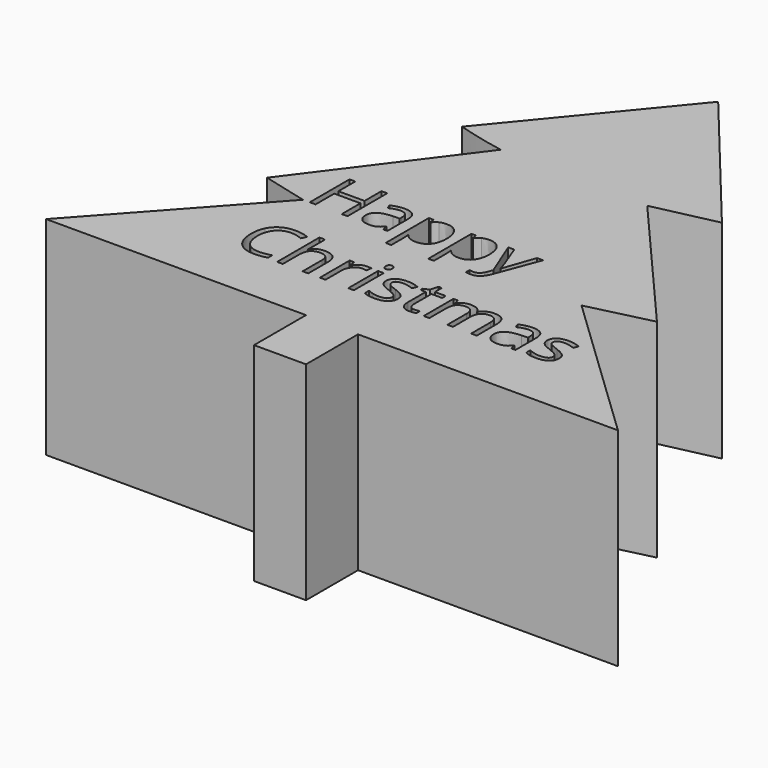
from build123d import *

# Parameters (mm, degrees)
F1_DEPTH = 6.95914
F2_W     = 0.8686156983
F2_H     = 5.7321941552
F3_DEPTH = 25


with BuildPart() as f1:
    # F0 (on Top) → F1 (new body)
    with BuildSketch(Plane.XY):
        with BuildLine():
            Line((-12.3236204717, 43.3583846717), (-32.2978136329, 19.0763476119))
            Line((-32.2978136329, 19.0763476119), (-12.2978136329, 19.0763476119))
            Line((-12.2978136329, 19.0763476119), (-12.2978136329, 43.3583799146))
            ThreePointArc((-12.2978136329, 43.3583799146), (-12.3107170525, 43.3583811039), (-12.3236204717, 43.3583846717))
        make_face()
        Polygon((-12.2978136329, 43.3583799146), (-12.2978136329, 19.0763476119), (7.7021863671, 19.0763476119), align=None)
        with BuildLine():
            ThreePointArc((-32.2978136329, 19.0763476119), (-28.6304707138, 18.0904479885), (-24.9150584445, 17.3048820634))
            ThreePointArc((-24.9150584445, 17.3048820634), (-18.6324272302, 16.4455999422), (-12.2978136329, 16.1583869369))
            Line((-12.2978136329, 16.1583869369), (-12.2978136329, 19.0763476119))
            Line((-12.2978136329, 19.0763476119), (-32.2978136329, 19.0763476119))
        make_face()
        with BuildLine():
            Line((-12.2978136329, 19.0763476119), (-12.2978136329, 16.1583869369))
            ThreePointArc((-12.2978136329, 16.1583869369), (-7.1653753165, 16.3467970901), (-2.0605656712, 16.9110133104))
            Line((-2.0605656712, 16.9110133104), (7.7021863671, 19.0763476119))
            Line((7.7021863671, 19.0763476119), (-12.2978136329, 19.0763476119))
        make_face()
        with BuildLine():
            Line((-24.9150584445, 17.3048820634), (-42.2978136329, -5.9236523881))
            Line((-42.2978136329, -5.9236523881), (-12.2978136329, -5.9236523881))
            Line((-12.2978136329, -5.9236523881), (-12.2978136329, 16.1583869369))
            ThreePointArc((-12.2978136329, 16.1583869369), (-18.6324272302, 16.4455999422), (-24.9150584445, 17.3048820634))
        make_face()
        with BuildLine():
            Line((-12.2978136329, 16.1583869369), (-12.2978136329, -5.9236523881))
            Line((-12.2978136329, -5.9236523881), (17.7021863671, -5.9236523881))
            Line((17.7021863671, -5.9236523881), (-2.0605656712, 16.9110133104))
            ThreePointArc((-2.0605656712, 16.9110133104), (-7.1653753165, 16.3467970901), (-12.2978136329, 16.1583869369))
        make_face()
        with BuildLine():
            Line((-42.2978136329, -5.9236523881), (-35.339471558, -7.7121023845))
            ThreePointArc((-35.339471558, -7.7121023845), (-23.8873413462, -9.60026092), (-12.2978136329, -10.2321441568))
            Line((-12.2978136329, -10.2321441568), (-12.2978136329, -5.9236523881))
            Line((-12.2978136329, -5.9236523881), (-42.2978136329, -5.9236523881))
        make_face()
        with BuildLine():
            Line((-12.2978136329, -5.9236523881), (-12.2978136329, -10.2321441568))
            ThreePointArc((-12.2978136329, -10.2321441568), (-2.1098095313, -9.7441780676), (7.9849217698, -8.2847472074))
            Line((7.9849217698, -8.2847472074), (17.7021863671, -5.9236523881))
            Line((17.7021863671, -5.9236523881), (-12.2978136329, -5.9236523881))
        make_face()
        with BuildLine():
            Line((-56.2978136329, -30.9236523881), (-16.2978136329, -30.9236523881))
            Line((-16.2978136329, -30.9236523881), (-12.2978136329, -30.9236523881))
            Line((-12.2978136329, -30.9236523881), (-12.2978136329, -10.2321441568))
            ThreePointArc((-12.2978136329, -10.2321441568), (-23.8873413462, -9.60026092), (-35.339471558, -7.7121023845))
            Line((-35.339471558, -7.7121023845), (-56.2978136329, -30.9236523881))
        make_face()
        with BuildLine():
            Line((-12.2978136329, -30.9236523881), (-8.2978136329, -30.9236523881))
            Line((-8.2978136329, -30.9236523881), (31.7021863671, -30.9236523881))
            Line((31.7021863671, -30.9236523881), (7.9849217698, -8.2847472074))
            ThreePointArc((7.9849217698, -8.2847472074), (-2.1098095313, -9.7441780676), (-12.2978136329, -10.2321441568))
            Line((-12.2978136329, -10.2321441568), (-12.2978136329, -30.9236523881))
        make_face()
        Polygon((-16.2978136329, -30.9236523881), (-16.2978136329, -40.9236523881), (-8.2978136329, -40.9236523881), (-8.2978136329, -30.9236523881), (-12.2978136329, -30.9236523881), align=None)
    extrude(amount=F1_DEPTH)

    # F2 (on face) → F3 (join)
    with BuildSketch(Plane.XY.offset(6.95914)):
        with BuildLine():
            Line((-2.0605656712, 16.9110133104), (7.7021863671, 19.0763476119))
            Line((7.7021863671, 19.0763476119), (-12.2978136329, 43.3583799146))
            ThreePointArc((-12.2978136329, 43.3583799146), (-12.3107170525, 43.3583811039), (-12.3236204717, 43.3583846717))
            Line((-12.3236204717, 43.3583846717), (-32.2978136329, 19.0763476119))
            ThreePointArc((-32.2978136329, 19.0763476119), (-28.6304707138, 18.0904479885), (-24.9150584445, 17.3048820634))
            Line((-24.9150584445, 17.3048820634), (-42.2978136329, -5.9236523881))
            Line((-42.2978136329, -5.9236523881), (-35.339471558, -7.7121023845))
            Line((-35.339471558, -7.7121023845), (-56.2978136329, -30.9236523881))
            Line((-56.2978136329, -30.9236523881), (-16.2978136329, -30.9236523881))
            Line((-16.2978136329, -30.9236523881), (-16.2978136329, -40.9236523881))
            Line((-16.2978136329, -40.9236523881), (-8.2978136329, -40.9236523881))
            Line((-8.2978136329, -40.9236523881), (-8.2978136329, -30.9236523881))
            Line((-8.2978136329, -30.9236523881), (31.7021863671, -30.9236523881))
            Line((31.7021863671, -30.9236523881), (7.9849217698, -8.2847472074))
            Line((7.9849217698, -8.2847472074), (17.7021863671, -5.9236523881))
            Line((17.7021863671, -5.9236523881), (-2.0605656712, 16.9110133104))
        make_face()
        with BuildLine():
            add(Edge.make_bspline(
                [(-29.2775716368, -15.7254587685), (-30.1461873351, -15.3187658693), (-31.0148030333, -15.3187658693)],
                knots=[0, 0, 0, 1, 1, 1], degree=2))
            add(Edge.make_bspline(
                [(-31.0148030333, -15.3187658693), (-32.2750489308, -15.3187658693), (-33.0047530627, -16.1580929843)],
                knots=[0, 0, 0, 1, 1, 1], degree=2))
            add(Edge.make_bspline(
                [(-33.0047530627, -16.1580929843), (-33.7344571945, -16.9974200992), (-33.7344571945, -18.456828363)],
                knots=[0, 0, 0, 1, 1, 1], degree=2))
            add(Edge.make_bspline(
                [(-33.7344571945, -18.456828363), (-33.7344571945, -19.9564038266), (-33.0306943793, -20.7756473417)],
                knots=[0, 0, 0, 1, 1, 1], degree=2))
            add(Edge.make_bspline(
                [(-33.0306943793, -20.7756473417), (-32.326931564, -21.5948908567), (-31.0248448333, -21.5948908567)],
                knots=[0, 0, 0, 1, 1, 1], degree=2))
            add(Edge.make_bspline(
                [(-31.0248448333, -21.5948908567), (-30.2248481016, -21.5948908567), (-29.1989108703, -21.3070259239)],
                knots=[0, 0, 0, 1, 1, 1], degree=2))
            Line((-29.1989108703, -21.3070259239), (-29.1989108703, -22.0852654224))
            add(Edge.make_bspline(
                [(-29.1989108703, -22.0852654224), (-29.993886702, -22.3848457884), (-31.160409133, -22.3848457884)],
                knots=[0, 0, 0, 1, 1, 1], degree=2))
            add(Edge.make_bspline(
                [(-31.160409133, -22.3848457884), (-32.849105163, -22.3848457884), (-33.7670930445, -21.3589085572)],
                knots=[0, 0, 0, 1, 1, 1], degree=2))
            add(Edge.make_bspline(
                [(-33.7670930445, -21.3589085572), (-34.685080926, -20.3329713259), (-34.685080926, -18.4451129297)],
                knots=[0, 0, 0, 1, 1, 1], degree=2))
            add(Edge.make_bspline(
                [(-34.685080926, -18.4451129297), (-34.685080926, -17.2635277987), (-34.2432417268, -16.3748285005)],
                knots=[0, 0, 0, 1, 1, 1], degree=2))
            add(Edge.make_bspline(
                [(-34.2432417268, -16.3748285005), (-33.8014025277, -15.4861292023), (-32.9670963127, -15.0049596199)],
                knots=[0, 0, 0, 1, 1, 1], degree=2))
            add(Edge.make_bspline(
                [(-32.9670963127, -15.0049596199), (-32.1327900977, -14.5237900375), (-31.0030876, -14.5237900375)],
                knots=[0, 0, 0, 1, 1, 1], degree=2))
            add(Edge.make_bspline(
                [(-31.0030876, -14.5237900375), (-29.8014188691, -14.5237900375), (-28.9010041375, -14.96228197)],
                knots=[0, 0, 0, 1, 1, 1], degree=2))
            Line((-28.9010041375, -14.96228197), (-29.2775716368, -15.7254587685))
        make_face(mode=Mode.SUBTRACT)
        with BuildLine():
            Line((-22.8692296163, -22.2794068887), (-23.7378453146, -22.2794068887))
            Line((-23.7378453146, -22.2794068887), (-23.7378453146, -18.5706354294))
            add(Edge.make_bspline(
                [(-23.7378453146, -18.5706354294), (-23.7378453146, -17.8710566975), (-24.0566724639, -17.5254514149)],
                knots=[0, 0, 0, 1, 1, 1], degree=2))
            add(Edge.make_bspline(
                [(-24.0566724639, -17.5254514149), (-24.3754996133, -17.1798461322), (-25.0566683786, -17.1798461322)],
                knots=[0, 0, 0, 1, 1, 1], degree=2))
            add(Edge.make_bspline(
                [(-25.0566683786, -17.1798461322), (-25.9604303768, -17.1798461322), (-26.3763282593, -17.6718943312)],
                knots=[0, 0, 0, 1, 1, 1], degree=2))
            add(Edge.make_bspline(
                [(-26.3763282593, -17.6718943312), (-26.7922261418, -18.1639425302), (-26.7922261418, -19.2819295947)],
                knots=[0, 0, 0, 1, 1, 1], degree=2))
            Line((-26.7922261418, -19.2819295947), (-26.7922261418, -22.2794068887))
            Line((-26.7922261418, -22.2794068887), (-27.66084184, -22.2794068887))
            Line((-27.66084184, -22.2794068887), (-27.66084184, -14.140528005))
            Line((-27.66084184, -14.140528005), (-26.7922261418, -14.140528005))
            Line((-26.7922261418, -14.140528005), (-26.7922261418, -16.6041162667))
            add(Edge.make_bspline(
                [(-26.7922261418, -16.6041162667), (-26.7922261418, -17.0493027325), (-26.834066975, -17.3421885652)],
                knots=[0, 0, 0, 1, 1, 1], degree=2))
            Line((-26.834066975, -17.3421885652), (-26.7821843418, -17.3421885652))
            add(Edge.make_bspline(
                [(-26.7821843418, -17.3421885652), (-26.5261184423, -16.9288011327), (-26.0524802099, -16.6911451999)],
                knots=[0, 0, 0, 1, 1, 1], degree=2))
            add(Edge.make_bspline(
                [(-26.0524802099, -16.6911451999), (-25.5788419775, -16.453489267), (-24.9729867121, -16.453489267)],
                knots=[0, 0, 0, 1, 1, 1], degree=2))
            add(Edge.make_bspline(
                [(-24.9729867121, -16.453489267), (-23.9219449809, -16.453489267), (-23.3955872986, -16.953068816)],
                knots=[0, 0, 0, 1, 1, 1], degree=2))
            add(Edge.make_bspline(
                [(-23.3955872986, -16.953068816), (-22.8692296163, -17.452648365), (-22.8692296163, -18.5405100295)],
                knots=[0, 0, 0, 1, 1, 1], degree=2))
            Line((-22.8692296163, -18.5405100295), (-22.8692296163, -22.2794068887))
        make_face(mode=Mode.SUBTRACT)
        with BuildLine():
            add(Edge.make_bspline(
                [(-19.4600385231, -16.7455382831), (-19.0098311574, -16.4417738337), (-18.4709212251, -16.4417738337)],
                knots=[0, 0, 0, 1, 1, 1], degree=2))
            add(Edge.make_bspline(
                [(-18.4709212251, -16.4417738337), (-18.0893328259, -16.4417738337), (-17.7864051932, -16.5053719002)],
                knots=[0, 0, 0, 1, 1, 1], degree=2))
            Line((-17.7864051932, -16.5053719002), (-17.9069067929, -17.310389532))
            add(Edge.make_bspline(
                [(-17.9069067929, -17.310389532), (-18.2617170589, -17.2317287654), (-18.5345192917, -17.2317287654)],
                knots=[0, 0, 0, 1, 1, 1], degree=2))
            add(Edge.make_bspline(
                [(-18.5345192917, -17.2317287654), (-19.2307507569, -17.2317287654), (-19.7244725893, -17.7965800143)],
                knots=[0, 0, 0, 1, 1, 1], degree=2))
            add(Edge.make_bspline(
                [(-19.7244725893, -17.7965800143), (-20.2181944216, -18.3614312632), (-20.2181944216, -19.2032688282)],
                knots=[0, 0, 0, 1, 1, 1], degree=2))
            Line((-20.2181944216, -19.2032688282), (-20.2181944216, -22.2794068887))
            Line((-20.2181944216, -22.2794068887), (-21.0868101199, -22.2794068887))
            Line((-21.0868101199, -22.2794068887), (-21.0868101199, -16.5472127335))
            Line((-21.0868101199, -16.5472127335), (-20.3704950547, -16.5472127335))
            Line((-20.3704950547, -16.5472127335), (-20.2700770549, -17.6082962647))
            Line((-20.2700770549, -17.6082962647), (-20.2282362216, -17.6082962647))
            add(Edge.make_bspline(
                [(-20.2282362216, -17.6082962647), (-19.9102458889, -17.0493027325), (-19.4600385231, -16.7455382831)],
                knots=[0, 0, 0, 1, 1, 1], degree=2))
        make_face(mode=Mode.SUBTRACT)
        with Locations((-16.2792983795, -19.4133098111)):
            Rectangle(F2_W, F2_H, mode=Mode.SUBTRACT)
        with BuildLine():
            add(Edge.make_bspline(
                [(-10.6650953741, -19.7689568937), (-10.3069378415, -20.1455243929), (-10.3069378415, -20.7162333585)],
                knots=[0, 0, 0, 1, 1, 1], degree=2))
            add(Edge.make_bspline(
                [(-10.3069378415, -20.7162333585), (-10.3069378415, -21.5162300902), (-10.902751307, -21.9505379393)],
                knots=[0, 0, 0, 1, 1, 1], degree=2))
            add(Edge.make_bspline(
                [(-10.902751307, -21.9505379393), (-11.4985647724, -22.3848457884), (-12.576384637, -22.3848457884)],
                knots=[0, 0, 0, 1, 1, 1], degree=2))
            add(Edge.make_bspline(
                [(-12.576384637, -22.3848457884), (-13.7161289347, -22.3848457884), (-14.3537832334, -22.0233409892)],
                knots=[0, 0, 0, 1, 1, 1], degree=2))
            Line((-14.3537832334, -22.0233409892), (-14.3537832334, -21.2183233574))
            add(Edge.make_bspline(
                [(-14.3537832334, -21.2183233574), (-13.9403958009, -21.4275275237), (-13.4675943852, -21.5471923068)],
                knots=[0, 0, 0, 1, 1, 1], degree=2))
            add(Edge.make_bspline(
                [(-13.4675943852, -21.5471923068), (-12.9947929694, -21.6668570899), (-12.5546274037, -21.6668570899)],
                knots=[0, 0, 0, 1, 1, 1], degree=2))
            add(Edge.make_bspline(
                [(-12.5546274037, -21.6668570899), (-11.8751322717, -21.6668570899), (-11.5094433891, -21.4501215737)],
                knots=[0, 0, 0, 1, 1, 1], degree=2))
            add(Edge.make_bspline(
                [(-11.5094433891, -21.4501215737), (-11.1437545065, -21.2333860574), (-11.1437545065, -20.7881995916)],
                knots=[0, 0, 0, 1, 1, 1], degree=2))
            add(Edge.make_bspline(
                [(-11.1437545065, -20.7881995916), (-11.1437545065, -20.4534729257), (-11.4332930726, -20.2158169928)],
                knots=[0, 0, 0, 1, 1, 1], degree=2))
            add(Edge.make_bspline(
                [(-11.4332930726, -20.2158169928), (-11.7228316387, -19.9781610599), (-12.566342837, -19.6534761939)],
                knots=[0, 0, 0, 1, 1, 1], degree=2))
            add(Edge.make_bspline(
                [(-12.566342837, -19.6534761939), (-13.3663395687, -19.3555694612), (-13.7035766847, -19.1329762283)],
                knots=[0, 0, 0, 1, 1, 1], degree=2))
            add(Edge.make_bspline(
                [(-13.7035766847, -19.1329762283), (-14.0408138007, -18.9103829954), (-14.2056666837, -18.6283757793)],
                knots=[0, 0, 0, 1, 1, 1], degree=2))
            add(Edge.make_bspline(
                [(-14.2056666837, -18.6283757793), (-14.3705195667, -18.3463685632), (-14.3705195667, -17.954738364)],
                knots=[0, 0, 0, 1, 1, 1], degree=2))
            add(Edge.make_bspline(
                [(-14.3705195667, -17.954738364), (-14.3705195667, -17.2534859987), (-13.7998106012, -16.8476299162)],
                knots=[0, 0, 0, 1, 1, 1], degree=2))
            add(Edge.make_bspline(
                [(-13.7998106012, -16.8476299162), (-13.2291016356, -16.4417738337), (-12.236637071, -16.4417738337)],
                knots=[0, 0, 0, 1, 1, 1], degree=2))
            add(Edge.make_bspline(
                [(-12.236637071, -16.4417738337), (-11.3111178395, -16.4417738337), (-10.4257658079, -16.8183413329)],
                knots=[0, 0, 0, 1, 1, 1], degree=2))
            Line((-10.4257658079, -16.8183413329), (-10.735387974, -17.5246145982))
            add(Edge.make_bspline(
                [(-10.735387974, -17.5246145982), (-11.5973091389, -17.1698043322), (-12.2985615042, -17.1698043322)],
                knots=[0, 0, 0, 1, 1, 1], degree=2))
            add(Edge.make_bspline(
                [(-12.2985615042, -17.1698043322), (-12.9161322029, -17.1698043322), (-13.2299384523, -17.3631089818)],
                knots=[0, 0, 0, 1, 1, 1], degree=2))
            add(Edge.make_bspline(
                [(-13.2299384523, -17.3631089818), (-13.5437447017, -17.5564136315), (-13.5437447017, -17.8961611974)],
                knots=[0, 0, 0, 1, 1, 1], degree=2))
            add(Edge.make_bspline(
                [(-13.5437447017, -17.8961611974), (-13.5437447017, -18.127122597), (-13.4257535519, -18.2886282133)],
                knots=[0, 0, 0, 1, 1, 1], degree=2))
            add(Edge.make_bspline(
                [(-13.4257535519, -18.2886282133), (-13.3077624022, -18.4501338297), (-13.0466756027, -18.596576746)],
                knots=[0, 0, 0, 1, 1, 1], degree=2))
            add(Edge.make_bspline(
                [(-13.0466756027, -18.596576746), (-12.7855888032, -18.7430196624), (-12.0424956047, -19.0208427952)],
                knots=[0, 0, 0, 1, 1, 1], degree=2))
            add(Edge.make_bspline(
                [(-12.0424956047, -19.0208427952), (-11.0232529067, -19.3923893944), (-10.6650953741, -19.7689568937)],
                knots=[0, 0, 0, 1, 1, 1], degree=2))
        make_face(mode=Mode.SUBTRACT)
        with BuildLine():
            add(Edge.make_bspline(
                [(-16.6408031788, -15.4308993024), (-16.7872460952, -15.286966836), (-16.7872460952, -14.9940810033)],
                knots=[0, 0, 0, 1, 1, 1], degree=2))
            add(Edge.make_bspline(
                [(-16.7872460952, -14.9940810033), (-16.7872460952, -14.6961742705), (-16.6408031788, -14.5572627041)],
                knots=[0, 0, 0, 1, 1, 1], degree=2))
            add(Edge.make_bspline(
                [(-16.6408031788, -14.5572627041), (-16.4943602624, -14.4183511378), (-16.2734406629, -14.4183511378)],
                knots=[0, 0, 0, 1, 1, 1], degree=2))
            add(Edge.make_bspline(
                [(-16.2734406629, -14.4183511378), (-16.0642364966, -14.4183511378), (-15.9127726803, -14.5597731541)],
                knots=[0, 0, 0, 1, 1, 1], degree=2))
            add(Edge.make_bspline(
                [(-15.9127726803, -14.5597731541), (-15.7613088639, -14.7011951705), (-15.7613088639, -14.9940810033)],
                knots=[0, 0, 0, 1, 1, 1], degree=2))
            add(Edge.make_bspline(
                [(-15.7613088639, -14.9940810033), (-15.7613088639, -15.286966836), (-15.9127726803, -15.4308993024)],
                knots=[0, 0, 0, 1, 1, 1], degree=2))
            add(Edge.make_bspline(
                [(-15.9127726803, -15.4308993024), (-16.0642364966, -15.5748317688), (-16.2734406629, -15.5748317688)],
                knots=[0, 0, 0, 1, 1, 1], degree=2))
            add(Edge.make_bspline(
                [(-16.2734406629, -15.5748317688), (-16.4943602624, -15.5748317688), (-16.6408031788, -15.4308993024)],
                knots=[0, 0, 0, 1, 1, 1], degree=2))
        make_face(mode=Mode.SUBTRACT)
        with BuildLine():
            Line((-22.3470560174, -7.7121023845), (-22.9914048494, -7.7121023845))
            Line((-22.9914048494, -7.7121023845), (-23.1637890824, -6.8953693195))
            Line((-23.1637890824, -6.8953693195), (-23.2056299156, -6.8953693195))
            add(Edge.make_bspline(
                [(-23.2056299156, -6.8953693195), (-23.6340800481, -7.4342792518), (-24.0600197306, -7.625910268)],
                knots=[0, 0, 0, 1, 1, 1], degree=2))
            add(Edge.make_bspline(
                [(-24.0600197306, -7.625910268), (-24.4859594131, -7.8175412843), (-25.1252873451, -7.8175412843)],
                knots=[0, 0, 0, 1, 1, 1], degree=2))
            add(Edge.make_bspline(
                [(-25.1252873451, -7.8175412843), (-25.9771667101, -7.8175412843), (-26.4608467424, -7.3773757185)],
                knots=[0, 0, 0, 1, 1, 1], degree=2))
            add(Edge.make_bspline(
                [(-26.4608467424, -7.3773757185), (-26.9445267748, -6.9372101528), (-26.9445267748, -6.127171621)],
                knots=[0, 0, 0, 1, 1, 1], degree=2))
            add(Edge.make_bspline(
                [(-26.9445267748, -6.127171621), (-26.9445267748, -4.3916138579), (-24.1679690804, -4.3079321914)],
                knots=[0, 0, 0, 1, 1, 1], degree=2))
            Line((-24.1679690804, -4.3079321914), (-23.1955881157, -4.2761331581))
            Line((-23.1955881157, -4.2761331581), (-23.1955881157, -3.9196492588))
            add(Edge.make_bspline(
                [(-23.1955881157, -3.9196492588), (-23.1955881157, -3.2451750268), (-23.4851266817, -2.9238374275)],
                knots=[0, 0, 0, 1, 1, 1], degree=2))
            add(Edge.make_bspline(
                [(-23.4851266817, -2.9238374275), (-23.7746652478, -2.6024998281), (-24.4139931799, -2.6024998281)],
                knots=[0, 0, 0, 1, 1, 1], degree=2))
            add(Edge.make_bspline(
                [(-24.4139931799, -2.6024998281), (-25.1303082451, -2.6024998281), (-26.0340702433, -3.0409917606)],
                knots=[0, 0, 0, 1, 1, 1], degree=2))
            Line((-26.0340702433, -3.0409917606), (-26.3018515761, -2.3765593286))
            add(Edge.make_bspline(
                [(-26.3018515761, -2.3765593286), (-25.8784223436, -2.1472715624), (-25.3738218946, -2.0167281626)],
                knots=[0, 0, 0, 1, 1, 1], degree=2))
            add(Edge.make_bspline(
                [(-25.3738218946, -2.0167281626), (-24.8692214456, -1.8861847629), (-24.3604369133, -1.8861847629)],
                knots=[0, 0, 0, 1, 1, 1], degree=2))
            add(Edge.make_bspline(
                [(-24.3604369133, -1.8861847629), (-23.3361733154, -1.8861847629), (-22.8416146664, -2.340576212)],
                knots=[0, 0, 0, 1, 1, 1], degree=2))
            add(Edge.make_bspline(
                [(-22.8416146664, -2.340576212), (-22.3470560174, -2.7949676611), (-22.3470560174, -3.799147659)],
                knots=[0, 0, 0, 1, 1, 1], degree=2))
            Line((-22.3470560174, -3.799147659), (-22.3470560174, -7.7121023845))
        make_face(mode=Mode.SUBTRACT)
        Polygon((-28.4825958051, -0.0652716999), (-28.4825958051, -7.7121023845), (-29.3712951033, -7.7121023845), (-29.3712951033, -4.1137907251), (-33.3997305285, -4.1137907251), (-33.3997305285, -7.7121023845), (-34.2884298267, -7.7121023845), (-34.2884298267, -0.0652716999), (-33.3997305285, -0.0652716999), (-33.3997305285, -3.3188148933), (-29.3712951033, -3.3188148933), (-29.3712951033, -0.0652716999), align=None, mode=Mode.SUBTRACT)
        with BuildLine():
            add(Edge.make_bspline(
                [(-16.1420604465, -7.0351177026), (-16.7721833952, -7.8175412843), (-17.891844093, -7.8175412843)],
                knots=[0, 0, 0, 1, 1, 1], degree=2))
            add(Edge.make_bspline(
                [(-17.891844093, -7.8175412843), (-18.4525112585, -7.8175412843), (-18.9152708742, -7.6108475681)],
                knots=[0, 0, 0, 1, 1, 1], degree=2))
            add(Edge.make_bspline(
                [(-18.9152708742, -7.6108475681), (-19.37803049, -7.4041538518), (-19.6909999227, -6.974030086)],
                knots=[0, 0, 0, 1, 1, 1], degree=2))
            Line((-19.6909999227, -6.974030086), (-19.7545979892, -6.974030086))
            add(Edge.make_bspline(
                [(-19.7545979892, -6.974030086), (-19.6909999227, -7.476120085), (-19.6909999227, -7.9263274508)],
                knots=[0, 0, 0, 1, 1, 1], degree=2))
            Line((-19.6909999227, -7.9263274508), (-19.6909999227, -10.286150446))
            Line((-19.6909999227, -10.286150446), (-20.5596156209, -10.286150446))
            Line((-20.5596156209, -10.286150446), (-20.5596156209, -1.9799082294))
            Line((-20.5596156209, -1.9799082294), (-19.8533423557, -1.9799082294))
            Line((-19.8533423557, -1.9799082294), (-19.7328407559, -2.7648422611))
            Line((-19.7328407559, -2.7648422611), (-19.6909999227, -2.7648422611))
            add(Edge.make_bspline(
                [(-19.6909999227, -2.7648422611), (-19.3562732567, -2.2928776621), (-18.9119236076, -2.0836734958)],
                knots=[0, 0, 0, 1, 1, 1], degree=2))
            add(Edge.make_bspline(
                [(-18.9119236076, -2.0836734958), (-18.4675739585, -1.8744693296), (-17.891844093, -1.8744693296)],
                knots=[0, 0, 0, 1, 1, 1], degree=2))
            add(Edge.make_bspline(
                [(-17.891844093, -1.8744693296), (-16.7520997952, -1.8744693296), (-16.1320186465, -2.6543824613)],
                knots=[0, 0, 0, 1, 1, 1], degree=2))
            add(Edge.make_bspline(
                [(-16.1320186465, -2.6543824613), (-15.5119374977, -3.4342955931), (-15.5119374977, -4.8401475903)],
                knots=[0, 0, 0, 1, 1, 1], degree=2))
            add(Edge.make_bspline(
                [(-15.5119374977, -4.8401475903), (-15.5119374977, -6.2526941208), (-16.1420604465, -7.0351177026)],
                knots=[0, 0, 0, 1, 1, 1], degree=2))
        make_face(mode=Mode.SUBTRACT)
        with BuildLine():
            add(Edge.make_bspline(
                [(-7.71782708, -21.3898707738), (-7.4718029805, -21.6668570899), (-7.043352848, -21.6668570899)],
                knots=[0, 0, 0, 1, 1, 1], degree=2))
            add(Edge.make_bspline(
                [(-7.043352848, -21.6668570899), (-6.8123914485, -21.6668570899), (-6.5981663823, -21.6333844233)],
                knots=[0, 0, 0, 1, 1, 1], degree=2))
            add(Edge.make_bspline(
                [(-6.5981663823, -21.6333844233), (-6.383941316, -21.5999117567), (-6.2584188163, -21.5630918234)],
                knots=[0, 0, 0, 1, 1, 1], degree=2))
            Line((-6.2584188163, -21.5630918234), (-6.2584188163, -22.2275242554))
            add(Edge.make_bspline(
                [(-6.2584188163, -22.2275242554), (-6.399004016, -22.2944695886), (-6.6734798821, -22.3396576885)],
                knots=[0, 0, 0, 1, 1, 1], degree=2))
            add(Edge.make_bspline(
                [(-6.6734798821, -22.3396576885), (-6.9479557482, -22.3848457884), (-7.1688753478, -22.3848457884)],
                knots=[0, 0, 0, 1, 1, 1], degree=2))
            add(Edge.make_bspline(
                [(-7.1688753478, -22.3848457884), (-8.8307932445, -22.3848457884), (-8.8307932445, -20.632551692)],
                knots=[0, 0, 0, 1, 1, 1], degree=2))
            Line((-8.8307932445, -20.632551692), (-8.8307932445, -17.2216869655))
            Line((-8.8307932445, -17.2216869655), (-9.6525472095, -17.2216869655))
            Line((-9.6525472095, -17.2216869655), (-9.6525472095, -16.803278633))
            Line((-9.6525472095, -16.803278633), (-8.8307932445, -16.4417738337))
            Line((-8.8307932445, -16.4417738337), (-8.4659411785, -15.2183478695))
            Line((-8.4659411785, -15.2183478695), (-7.9638511795, -15.2183478695))
            Line((-7.9638511795, -15.2183478695), (-7.9638511795, -16.5472127335))
            Line((-7.9638511795, -16.5472127335), (-6.3002596495, -16.5472127335))
            Line((-6.3002596495, -16.5472127335), (-6.3002596495, -17.2216869655))
            Line((-6.3002596495, -17.2216869655), (-7.9638511795, -17.2216869655))
            Line((-7.9638511795, -17.2216869655), (-7.9638511795, -20.5957317587))
            add(Edge.make_bspline(
                [(-7.9638511795, -20.5957317587), (-7.9638511795, -21.1128844577), (-7.71782708, -21.3898707738)],
                knots=[0, 0, 0, 1, 1, 1], degree=2))
        make_face(mode=Mode.SUBTRACT)
        with BuildLine():
            Line((3.060371565, -22.2794068887), (2.1934295001, -22.2794068887))
            Line((2.1934295001, -22.2794068887), (2.1934295001, -18.5505518295))
            add(Edge.make_bspline(
                [(2.1934295001, -18.5505518295), (2.1934295001, -17.8643621642), (1.9005436673, -17.5221041482)],
                knots=[0, 0, 0, 1, 1, 1], degree=2))
            add(Edge.make_bspline(
                [(1.9005436673, -17.5221041482), (1.6076578346, -17.1798461322), (0.9900871358, -17.1798461322)],
                knots=[0, 0, 0, 1, 1, 1], degree=2))
            add(Edge.make_bspline(
                [(0.9900871358, -17.1798461322), (0.1800486041, -17.1798461322), (-0.2073975118, -17.6451161979)],
                knots=[0, 0, 0, 1, 1, 1], degree=2))
            add(Edge.make_bspline(
                [(-0.2073975118, -17.6451161979), (-0.5948436276, -18.1103862637), (-0.5948436276, -19.0777463284)],
                knots=[0, 0, 0, 1, 1, 1], degree=2))
            Line((-0.5948436276, -19.0777463284), (-0.5948436276, -22.2794068887))
            Line((-0.5948436276, -22.2794068887), (-1.4634593259, -22.2794068887))
            Line((-1.4634593259, -22.2794068887), (-1.4634593259, -18.5505518295))
            add(Edge.make_bspline(
                [(-1.4634593259, -18.5505518295), (-1.4634593259, -17.8643621642), (-1.7563451587, -17.5221041482)],
                knots=[0, 0, 0, 1, 1, 1], degree=2))
            add(Edge.make_bspline(
                [(-1.7563451587, -17.5221041482), (-2.0492309914, -17.1798461322), (-2.6718225901, -17.1798461322)],
                knots=[0, 0, 0, 1, 1, 1], degree=2))
            add(Edge.make_bspline(
                [(-2.6718225901, -17.1798461322), (-3.4868820218, -17.1798461322), (-3.8659599711, -17.6685470646)],
                knots=[0, 0, 0, 1, 1, 1], degree=2))
            add(Edge.make_bspline(
                [(-3.8659599711, -17.6685470646), (-4.2450379203, -18.1572479969), (-4.2450379203, -19.2718877947)],
                knots=[0, 0, 0, 1, 1, 1], degree=2))
            Line((-4.2450379203, -19.2718877947), (-4.2450379203, -22.2794068887))
            Line((-4.2450379203, -22.2794068887), (-5.1136536186, -22.2794068887))
            Line((-5.1136536186, -22.2794068887), (-5.1136536186, -16.5472127335))
            Line((-5.1136536186, -16.5472127335), (-4.4073803533, -16.5472127335))
            Line((-4.4073803533, -16.5472127335), (-4.2667951536, -17.3321467652))
            Line((-4.2667951536, -17.3321467652), (-4.2249543204, -17.3321467652))
            add(Edge.make_bspline(
                [(-4.2249543204, -17.3321467652), (-3.9789302209, -16.9137384327), (-3.5312333051, -16.6777561332)],
                knots=[0, 0, 0, 1, 1, 1], degree=2))
            add(Edge.make_bspline(
                [(-3.5312333051, -16.6777561332), (-3.0835363893, -16.4417738337), (-2.5295637571, -16.4417738337)],
                knots=[0, 0, 0, 1, 1, 1], degree=2))
            add(Edge.make_bspline(
                [(-2.5295637571, -16.4417738337), (-1.1856361931, -16.4417738337), (-0.7722487606, -17.4158284317)],
                knots=[0, 0, 0, 1, 1, 1], degree=2))
            Line((-0.7722487606, -17.4158284317), (-0.7304079274, -17.4158284317))
            add(Edge.make_bspline(
                [(-0.7304079274, -17.4158284317), (-0.4743420279, -16.965621066), (0.0118484545, -16.7036974498)],
                knots=[0, 0, 0, 1, 1, 1], degree=2))
            add(Edge.make_bspline(
                [(0.0118484545, -16.7036974498), (0.4980389368, -16.4417738337), (1.1206305356, -16.4417738337)],
                knots=[0, 0, 0, 1, 1, 1], degree=2))
            add(Edge.make_bspline(
                [(1.1206305356, -16.4417738337), (2.0930115003, -16.4417738337), (2.5766915327, -16.9413533827)],
                knots=[0, 0, 0, 1, 1, 1], degree=2))
            add(Edge.make_bspline(
                [(2.5766915327, -16.9413533827), (3.060371565, -17.4409329317), (3.060371565, -18.5405100295)],
                knots=[0, 0, 0, 1, 1, 1], degree=2))
            Line((3.060371565, -18.5405100295), (3.060371565, -22.2794068887))
        make_face(mode=Mode.SUBTRACT)
        with BuildLine():
            Line((9.0185062197, -22.2794068887), (8.3741573877, -22.2794068887))
            Line((8.3741573877, -22.2794068887), (8.2017731547, -21.4626738236))
            Line((8.2017731547, -21.4626738236), (8.1599323215, -21.4626738236))
            add(Edge.make_bspline(
                [(8.1599323215, -21.4626738236), (7.731482189, -22.0015837559), (7.3055425065, -22.1932147722)],
                knots=[0, 0, 0, 1, 1, 1], degree=2))
            add(Edge.make_bspline(
                [(7.3055425065, -22.1932147722), (6.879602824, -22.3848457884), (6.240274892, -22.3848457884)],
                knots=[0, 0, 0, 1, 1, 1], degree=2))
            add(Edge.make_bspline(
                [(6.240274892, -22.3848457884), (5.388395527, -22.3848457884), (4.9047154947, -21.9446802227)],
                knots=[0, 0, 0, 1, 1, 1], degree=2))
            add(Edge.make_bspline(
                [(4.9047154947, -21.9446802227), (4.4210354623, -21.5045146569), (4.4210354623, -20.6944761252)],
                knots=[0, 0, 0, 1, 1, 1], degree=2))
            add(Edge.make_bspline(
                [(4.4210354623, -20.6944761252), (4.4210354623, -18.958918362), (7.1975931567, -18.8752366955)],
                knots=[0, 0, 0, 1, 1, 1], degree=2))
            Line((7.1975931567, -18.8752366955), (8.1699741214, -18.8434376622))
            Line((8.1699741214, -18.8434376622), (8.1699741214, -18.4869537629))
            add(Edge.make_bspline(
                [(8.1699741214, -18.4869537629), (8.1699741214, -17.8124795309), (7.8804355554, -17.4911419316)],
                knots=[0, 0, 0, 1, 1, 1], degree=2))
            add(Edge.make_bspline(
                [(7.8804355554, -17.4911419316), (7.5908969893, -17.1698043322), (6.9515690572, -17.1698043322)],
                knots=[0, 0, 0, 1, 1, 1], degree=2))
            add(Edge.make_bspline(
                [(6.9515690572, -17.1698043322), (6.235253992, -17.1698043322), (5.3314919938, -17.6082962647)],
                knots=[0, 0, 0, 1, 1, 1], degree=2))
            Line((5.3314919938, -17.6082962647), (5.063710661, -16.9438638327))
            add(Edge.make_bspline(
                [(5.063710661, -16.9438638327), (5.4871398935, -16.7145760665), (5.9917403425, -16.5840326667)],
                knots=[0, 0, 0, 1, 1, 1], degree=2))
            add(Edge.make_bspline(
                [(5.9917403425, -16.5840326667), (6.4963407915, -16.453489267), (7.0051253238, -16.453489267)],
                knots=[0, 0, 0, 1, 1, 1], degree=2))
            add(Edge.make_bspline(
                [(7.0051253238, -16.453489267), (8.0293889217, -16.453489267), (8.5239475707, -16.9078807161)],
                knots=[0, 0, 0, 1, 1, 1], degree=2))
            add(Edge.make_bspline(
                [(8.5239475707, -16.9078807161), (9.0185062197, -17.3622721652), (9.0185062197, -18.3664521632)],
                knots=[0, 0, 0, 1, 1, 1], degree=2))
            Line((9.0185062197, -18.3664521632), (9.0185062197, -22.2794068887))
        make_face(mode=Mode.SUBTRACT)
        with BuildLine():
            add(Edge.make_bspline(
                [(-9.5780705263, -7.0351177026), (-10.208193475, -7.8175412843), (-11.3278541728, -7.8175412843)],
                knots=[0, 0, 0, 1, 1, 1], degree=2))
            add(Edge.make_bspline(
                [(-11.3278541728, -7.8175412843), (-11.8885213383, -7.8175412843), (-12.3512809541, -7.6108475681)],
                knots=[0, 0, 0, 1, 1, 1], degree=2))
            add(Edge.make_bspline(
                [(-12.3512809541, -7.6108475681), (-12.8140405698, -7.4041538518), (-13.1270100025, -6.974030086)],
                knots=[0, 0, 0, 1, 1, 1], degree=2))
            Line((-13.1270100025, -6.974030086), (-13.1906080691, -6.974030086))
            add(Edge.make_bspline(
                [(-13.1906080691, -6.974030086), (-13.1270100025, -7.476120085), (-13.1270100025, -7.9263274508)],
                knots=[0, 0, 0, 1, 1, 1], degree=2))
            Line((-13.1270100025, -7.9263274508), (-13.1270100025, -10.286150446))
            Line((-13.1270100025, -10.286150446), (-13.9956257008, -10.286150446))
            Line((-13.9956257008, -10.286150446), (-13.9956257008, -1.9799082294))
            Line((-13.9956257008, -1.9799082294), (-13.2893524355, -1.9799082294))
            Line((-13.2893524355, -1.9799082294), (-13.1688508358, -2.7648422611))
            Line((-13.1688508358, -2.7648422611), (-13.1270100025, -2.7648422611))
            add(Edge.make_bspline(
                [(-13.1270100025, -2.7648422611), (-12.7922833365, -2.2928776621), (-12.3479336874, -2.0836734958)],
                knots=[0, 0, 0, 1, 1, 1], degree=2))
            add(Edge.make_bspline(
                [(-12.3479336874, -2.0836734958), (-11.9035840383, -1.8744693296), (-11.3278541728, -1.8744693296)],
                knots=[0, 0, 0, 1, 1, 1], degree=2))
            add(Edge.make_bspline(
                [(-11.3278541728, -1.8744693296), (-10.1881098751, -1.8744693296), (-9.5680287263, -2.6543824613)],
                knots=[0, 0, 0, 1, 1, 1], degree=2))
            add(Edge.make_bspline(
                [(-9.5680287263, -2.6543824613), (-8.9479475776, -3.4342955931), (-8.9479475776, -4.8401475903)],
                knots=[0, 0, 0, 1, 1, 1], degree=2))
            add(Edge.make_bspline(
                [(-8.9479475776, -4.8401475903), (-8.9479475776, -6.2526941208), (-9.5780705263, -7.0351177026)],
                knots=[0, 0, 0, 1, 1, 1], degree=2))
        make_face(mode=Mode.SUBTRACT)
        with BuildLine():
            Line((-6.0291310501, -7.7439014178), (-8.3420923121, -1.9799082294))
            Line((-8.3420923121, -1.9799082294), (-7.4098785473, -1.9799082294))
            Line((-7.4098785473, -1.9799082294), (-6.1546535498, -5.2485141228))
            add(Edge.make_bspline(
                [(-6.1546535498, -5.2485141228), (-5.7429397507, -6.3681748206), (-5.6425217509, -6.8652439196)],
                knots=[0, 0, 0, 1, 1, 1], degree=2))
            Line((-5.6425217509, -6.8652439196), (-5.6006809176, -6.8652439196))
            add(Edge.make_bspline(
                [(-5.6006809176, -6.8652439196), (-5.5337355844, -6.5974625868), (-5.3161632515, -5.9514401214)],
                knots=[0, 0, 0, 1, 1, 1], degree=2))
            add(Edge.make_bspline(
                [(-5.3161632515, -5.9514401214), (-5.0985909186, -5.305417656), (-3.8952485544, -1.9799082294)],
                knots=[0, 0, 0, 1, 1, 1], degree=2))
            Line((-3.8952485544, -1.9799082294), (-2.9647084229, -1.9799082294))
            Line((-2.9647084229, -1.9799082294), (-5.4282966846, -8.5070782163))
            add(Edge.make_bspline(
                [(-5.4282966846, -8.5070782163), (-5.7948223839, -9.474438281), (-6.2835233162, -9.8802943635)],
                knots=[0, 0, 0, 1, 1, 1], degree=2))
            add(Edge.make_bspline(
                [(-6.2835233162, -9.8802943635), (-6.7722242486, -10.286150446), (-7.4835184138, -10.286150446)],
                knots=[0, 0, 0, 1, 1, 1], degree=2))
            add(Edge.make_bspline(
                [(-7.4835184138, -10.286150446), (-7.8818431464, -10.286150446), (-8.2684524456, -10.1957742462)],
                knots=[0, 0, 0, 1, 1, 1], degree=2))
            Line((-8.2684524456, -10.1957742462), (-8.2684524456, -9.5012164143))
            add(Edge.make_bspline(
                [(-8.2684524456, -9.5012164143), (-7.9805875128, -9.5631408475), (-7.6257772469, -9.5631408475)],
                knots=[0, 0, 0, 1, 1, 1], degree=2))
            add(Edge.make_bspline(
                [(-7.6257772469, -9.5631408475), (-6.7303834153, -9.5631408475), (-6.3487950161, -8.5589608495)],
                knots=[0, 0, 0, 1, 1, 1], degree=2))
            Line((-6.3487950161, -8.5589608495), (-6.0291310501, -7.7439014178))
        make_face(mode=Mode.SUBTRACT)
        with BuildLine():
            add(Edge.make_bspline(
                [(14.1448451095, -19.7689568937), (14.5030026421, -20.1455243929), (14.5030026421, -20.7162333585)],
                knots=[0, 0, 0, 1, 1, 1], degree=2))
            add(Edge.make_bspline(
                [(14.5030026421, -20.7162333585), (14.5030026421, -21.5162300902), (13.9071891766, -21.9505379393)],
                knots=[0, 0, 0, 1, 1, 1], degree=2))
            add(Edge.make_bspline(
                [(13.9071891766, -21.9505379393), (13.3113757111, -22.3848457884), (12.2335558466, -22.3848457884)],
                knots=[0, 0, 0, 1, 1, 1], degree=2))
            add(Edge.make_bspline(
                [(12.2335558466, -22.3848457884), (11.0938115489, -22.3848457884), (10.4561572502, -22.0233409892)],
                knots=[0, 0, 0, 1, 1, 1], degree=2))
            Line((10.4561572502, -22.0233409892), (10.4561572502, -21.2183233574))
            add(Edge.make_bspline(
                [(10.4561572502, -21.2183233574), (10.8695446827, -21.4275275237), (11.3423460984, -21.5471923068)],
                knots=[0, 0, 0, 1, 1, 1], degree=2))
            add(Edge.make_bspline(
                [(11.3423460984, -21.5471923068), (11.8151475141, -21.6668570899), (12.2553130799, -21.6668570899)],
                knots=[0, 0, 0, 1, 1, 1], degree=2))
            add(Edge.make_bspline(
                [(12.2553130799, -21.6668570899), (12.9348082119, -21.6668570899), (13.3004970945, -21.4501215737)],
                knots=[0, 0, 0, 1, 1, 1], degree=2))
            add(Edge.make_bspline(
                [(13.3004970945, -21.4501215737), (13.6661859771, -21.2333860574), (13.6661859771, -20.7881995916)],
                knots=[0, 0, 0, 1, 1, 1], degree=2))
            add(Edge.make_bspline(
                [(13.6661859771, -20.7881995916), (13.6661859771, -20.4534729257), (13.376647411, -20.2158169928)],
                knots=[0, 0, 0, 1, 1, 1], degree=2))
            add(Edge.make_bspline(
                [(13.376647411, -20.2158169928), (13.0871088449, -19.9781610599), (12.2435976466, -19.6534761939)],
                knots=[0, 0, 0, 1, 1, 1], degree=2))
            add(Edge.make_bspline(
                [(12.2435976466, -19.6534761939), (11.4436009149, -19.3555694612), (11.1063637989, -19.1329762283)],
                knots=[0, 0, 0, 1, 1, 1], degree=2))
            add(Edge.make_bspline(
                [(11.1063637989, -19.1329762283), (10.7691266829, -18.9103829954), (10.6042737999, -18.6283757793)],
                knots=[0, 0, 0, 1, 1, 1], degree=2))
            add(Edge.make_bspline(
                [(10.6042737999, -18.6283757793), (10.4394209169, -18.3463685632), (10.4394209169, -17.954738364)],
                knots=[0, 0, 0, 1, 1, 1], degree=2))
            add(Edge.make_bspline(
                [(10.4394209169, -17.954738364), (10.4394209169, -17.2534859987), (11.0101298824, -16.8476299162)],
                knots=[0, 0, 0, 1, 1, 1], degree=2))
            add(Edge.make_bspline(
                [(11.0101298824, -16.8476299162), (11.5808388479, -16.4417738337), (12.5733034126, -16.4417738337)],
                knots=[0, 0, 0, 1, 1, 1], degree=2))
            add(Edge.make_bspline(
                [(12.5733034126, -16.4417738337), (13.4988226441, -16.4417738337), (14.3841746756, -16.8183413329)],
                knots=[0, 0, 0, 1, 1, 1], degree=2))
            Line((14.3841746756, -16.8183413329), (14.0745525096, -17.5246145982))
            add(Edge.make_bspline(
                [(14.0745525096, -17.5246145982), (13.2126313447, -17.1698043322), (12.5113789794, -17.1698043322)],
                knots=[0, 0, 0, 1, 1, 1], degree=2))
            add(Edge.make_bspline(
                [(12.5113789794, -17.1698043322), (11.8938082806, -17.1698043322), (11.5800020313, -17.3631089818)],
                knots=[0, 0, 0, 1, 1, 1], degree=2))
            add(Edge.make_bspline(
                [(11.5800020313, -17.3631089818), (11.2661957819, -17.5564136315), (11.2661957819, -17.8961611974)],
                knots=[0, 0, 0, 1, 1, 1], degree=2))
            add(Edge.make_bspline(
                [(11.2661957819, -17.8961611974), (11.2661957819, -18.127122597), (11.3841869317, -18.2886282133)],
                knots=[0, 0, 0, 1, 1, 1], degree=2))
            add(Edge.make_bspline(
                [(11.3841869317, -18.2886282133), (11.5021780814, -18.4501338297), (11.7632648809, -18.596576746)],
                knots=[0, 0, 0, 1, 1, 1], degree=2))
            add(Edge.make_bspline(
                [(11.7632648809, -18.596576746), (12.0243516804, -18.7430196624), (12.7674448789, -19.0208427952)],
                knots=[0, 0, 0, 1, 1, 1], degree=2))
            add(Edge.make_bspline(
                [(12.7674448789, -19.0208427952), (13.7866875768, -19.3923893944), (14.1448451095, -19.7689568937)],
                knots=[0, 0, 0, 1, 1, 1], degree=2))
        make_face(mode=Mode.SUBTRACT)
    extrude(amount=F3_DEPTH)


solid = f1.part
